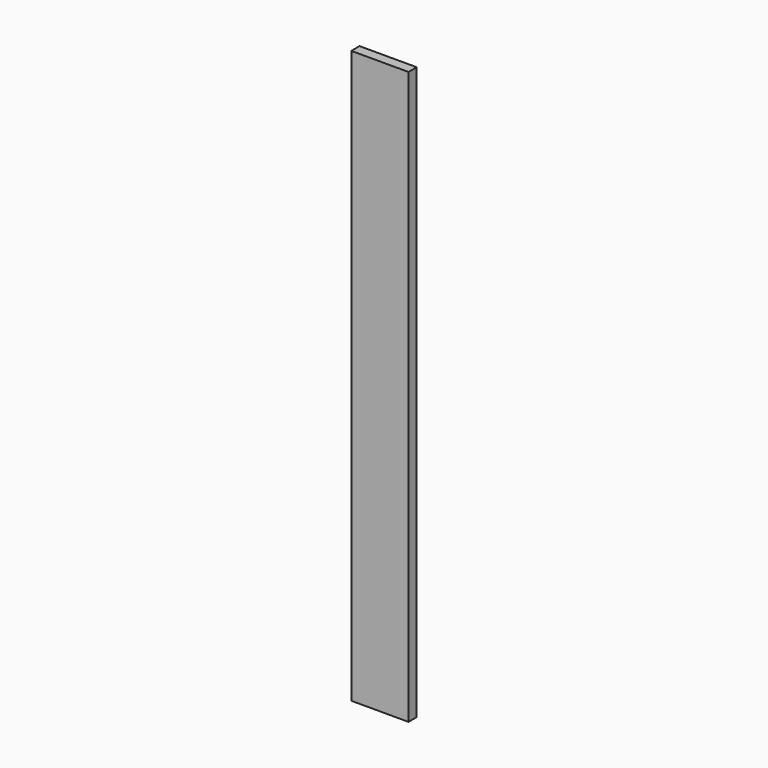
from build123d import *

# Parameters (mm, degrees)
F0_W     = 100
F0_H     = 1000
F1_DEPTH = 18


# Not quite as in the source:
# - a feature names something its author has since deleted; it is built from what else it names


with BuildPart() as f1:
    # F0 (on Front) → F1 (new body)
    with BuildSketch(Plane.XZ):
        with Locations((50, 500)):
            Rectangle(F0_W, F0_H)
    extrude(amount=F1_DEPTH)


solid = f1.part
